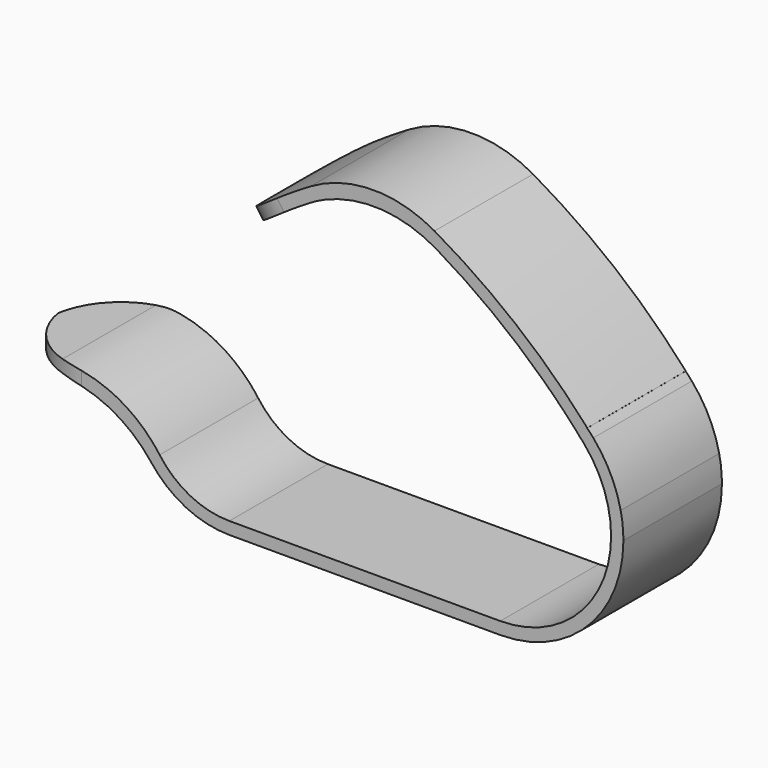
from build123d import *

# Parameters (mm, degrees)
F1_DEPTH    = 5
F2_R        = 5
F3_R        = 5
F4_R        = 5
F5_R        = 5
F6_R        = 2.49999
F7_T1_DEPTH = 15.5


# Not quite as in the source:
# - a fillet or chamfer that OpenCascade refuses, or shapes differently, is made with other operations: its cross-section is extruded or revolved along the edge and cut away or added
# - a fillet or chamfer is up to 0.001 mm smaller than in the source, because OpenCascade refuses the exact size
# - ends of sketch curves that miss each other by under 0.0002 mm in the source are joined


with BuildPart() as f1:
    # F0 (on Front) → F1 (new body)
    with BuildSketch(Plane.XZ):
        with BuildLine():
            ThreePointArc((8.5340575526, 1.5524331459), (5.288604189, 4.5896124098), (1.5539747452, 7))
            Line((1.5539747452, 7), (0.4354276506, 7))
            ThreePointArc((0.4354276506, 7), (3.7532215697, 5.0934578086), (6.7313555625, 2.6906724375))
            ThreePointArc((6.7313555625, 2.6906724375), (7.6907583635, 2.2142400773), (8.526661649, 1.544383954))
            Line((8.526661649, 1.544383954), (8.5340575526, 1.5524331459))
        make_face()
        with BuildLine():
            Line((0.4354276506, 7), (1.5539747452, 7))
            ThreePointArc((1.5539747452, 7), (0.9960319704, 7.2841112302), (0.4311083103, 7.5540752821))
            ThreePointArc((0.4311083103, 7.5540752821), (0.1227273169, 7.4207378189), (-0.1837962437, 7.2831841097))
            ThreePointArc((-0.1837962437, 7.2831841097), (0.1268056153, 7.1437566434), (0.4354276506, 7))
        make_face()
        with BuildLine():
            ThreePointArc((-0.1837962437, 7.2831841097), (0.1227273169, 7.4207378189), (0.4311083103, 7.5540752821))
            ThreePointArc((0.4311083103, 7.5540752821), (0.1226739578, 7.6941799666), (-0.1876416897, 7.830066947))
            ThreePointArc((-0.1876416897, 7.830066947), (-0.4960575858, 7.6899267332), (-0.8025462438, 7.5456202987))
            ThreePointArc((-0.8025462438, 7.5456202987), (-0.4922657174, 7.4165371782), (-0.1837962437, 7.2831841097))
        make_face()
        with BuildLine():
            ThreePointArc((9.8891323912, -0.952916211), (9.474622014, 0.231088934), (8.7784454506, 1.2746526497))
            ThreePointArc((8.7784454506, 1.2746526497), (8.6550425686, 1.4118417052), (8.526661649, 1.544383954))
            Line((8.526661649, 1.544383954), (8.1941180403, 1.1824664061))
            ThreePointArc((8.1941180403, 1.1824664061), (8.2977627182, 1.0651806637), (8.4006513445, 0.9472311186))
            ThreePointArc((8.4006513445, 0.9472311186), (9.1684512833, 0.0156127298), (9.8891323912, -0.952916211))
        make_face()
        with BuildLine():
            ThreePointArc((-5.7758389138, 3.7449434933), (-3.3782514437, 5.5249211523), (-0.7819293264, 7))
            Line((-0.7819293264, 7), (-1.874342087, 7))
            ThreePointArc((-1.874342087, 7), (-4.0392081747, 5.6857592036), (-6.0600011216, 4.1592370405))
            Line((-6.0600011216, 4.1592370405), (-5.7758389138, 3.7449434933))
        make_face()
        with BuildLine():
            Line((-1.874342087, 7), (-0.7819293264, 7))
            ThreePointArc((-0.7819293264, 7), (-0.4838189836, 7.143611709), (-0.1837962437, 7.2831841097))
            ThreePointArc((-0.1837962437, 7.2831841097), (-0.4922657174, 7.4165371782), (-0.8025462438, 7.5456202987))
            ThreePointArc((-0.8025462438, 7.5456202987), (-1.341725683, 7.2792562383), (-1.874342087, 7))
        make_face()
        with BuildLine():
            ThreePointArc((8.526661649, 1.544383954), (7.6907583635, 2.2142400773), (6.7313555625, 2.6906724375))
            ThreePointArc((6.7313555625, 2.6906724375), (7.4790116412, 1.9523538866), (8.1941180403, 1.1824664061))
            Line((8.1941180403, 1.1824664061), (8.526661649, 1.544383954))
        make_face()
        with BuildLine():
            ThreePointArc((5, -7), (8.5355339059, -5.5355339059), (10, -2))
            ThreePointArc((10, -2), (9.9722058463, -1.4735315565), (9.8891323912, -0.952916211))
            ThreePointArc((9.8891323912, -0.952916211), (9.1684512833, 0.0156127298), (8.4006513445, 0.9472311186))
            ThreePointArc((8.4006513445, 0.9472311186), (9.2162011355, -0.4272164851), (9.5, -2))
            ThreePointArc((9.5, -2), (8.1819805153, -5.1819805153), (5, -6.5))
            Line((5, -6.5), (5, -7))
        make_face()
        with BuildLine():
            Line((4.8047364689, -6.5), (2.8205505282, -6.5))
            ThreePointArc((2.8205505282, -6.5), (3.7870014268, -6.8506323775), (4.8047364689, -6.9961857605))
            Line((4.8047364689, -6.9961857605), (4.8047364689, -6.5))
        make_face()
        with BuildLine():
            ThreePointArc((4.8047364689, -6.9961857605), (3.7870014268, -6.8506323775), (2.8205505282, -6.5))
            Line((2.8205505282, -6.5), (-4.0635083269, -6.5))
            ThreePointArc((-4.0635083269, -6.5), (-5, -6.8729833462), (-6, -7))
            Line((-6, -7), (4.8047364689, -7))
            Line((4.8047364689, -7), (4.8047364689, -6.9961857605))
        make_face()
        with BuildLine():
            ThreePointArc((8.4006513445, 0.9472311186), (8.2977627182, 1.0651806637), (8.1941180403, 1.1824664061))
            Line((8.1941180403, 1.1824664061), (8.1880677147, 1.1758816487))
            ThreePointArc((8.1880677147, 1.1758816487), (8.2963182158, 1.0633782366), (8.4006513445, 0.9472311186))
        make_face()
        with BuildLine():
            ThreePointArc((4.8047364689, -6.9961857605), (4.9023496096, -6.9990463492), (5, -7))
            Line((5, -7), (5, -6.5))
            Line((5, -6.5), (4.8047364689, -6.5))
            Line((4.8047364689, -6.5), (4.8047364689, -6.9961857605))
        make_face()
        with BuildLine():
            ThreePointArc((-6, -7), (-5, -6.8729833462), (-4.0635083269, -6.5))
            Line((-4.0635083269, -6.5), (-6, -6.5))
            Line((-6, -6.5), (-6, -7))
        make_face()
        with BuildLine():
            Line((-12.1979728804, -3.5), (-11.6333076528, -3.5))
            ThreePointArc((-11.6333076528, -3.5), (-11.4981121732, -3.2492054316), (-11.3600093633, -3))
            Line((-11.3600093633, -3), (-11.9317121995, -3))
            ThreePointArc((-11.9317121995, -3), (-12.0662587747, -3.2492458247), (-12.1979728804, -3.5))
        make_face()
        with BuildLine():
            ThreePointArc((-11.3600093633, -3), (-11.4981121732, -3.2492054316), (-11.6333076528, -3.5))
            Line((-11.6333076528, -3.5), (-10, -3.5))
            Line((-10, -3.5), (-10, -3))
            Line((-10, -3), (-11.3600093633, -3))
        make_face()
        with BuildLine():
            ThreePointArc((-9.9686269666, -3.5), (-9.9921490369, -3.2504916502), (-10, -3))
            Line((-10, -3), (-10, -3.5))
            Line((-10, -3.5), (-9.9686269666, -3.5))
        make_face()
        with BuildLine():
            Line((-9.5, -3), (-10, -3))
            ThreePointArc((-10, -3), (-9.9921490369, -3.2504916502), (-9.9686269666, -3.5))
            Line((-9.9686269666, -3.5), (-9.4641016151, -3.5))
            ThreePointArc((-9.4641016151, -3.5), (-9.491013868, -3.2506435188), (-9.5, -3))
        make_face()
        with BuildLine():
            ThreePointArc((-9.9686269666, -3.5), (-8.6457513111, -6), (-6, -7))
            Line((-6, -7), (-6, -6.5))
            ThreePointArc((-6, -6.5), (-8.2912878475, -5.6457513111), (-9.4641016151, -3.5))
            Line((-9.4641016151, -3.5), (-9.9686269666, -3.5))
        make_face()
        with BuildLine():
            Line((-15, -3.5), (-12.1979728804, -3.5))
            ThreePointArc((-12.1979728804, -3.5), (-12.0662587747, -3.2492458247), (-11.9317121995, -3))
            Line((-11.9317121995, -3), (-15, -3))
            Line((-15, -3), (-15, -3.5))
        make_face()
    extrude(amount=F1_DEPTH)

    # F2
    f2_edges = [f1.edges().sort_by_distance(p)[0] for p in [
        (-9.968627, -2.5, -3.5),
    ]]
    fillet(f2_edges, radius=F2_R)

    # F3
    f3_edges = [f1.edges().sort_by_distance(p)[0] for p in [
        (-9.5, -2.5, -3),
    ]]
    fillet(f3_edges, radius=F3_R)

    # F4
    f4_edges = [f1.edges().sort_by_distance(p)[0] for p in [
        (-0.183796, -2.5, 7.283184),
    ]]
    fillet(f4_edges, radius=F4_R)

    # F5
    f5_edges = [f1.edges().sort_by_distance(p)[0] for p in [
        (-0.187642, -2.5, 7.830067),
    ]]
    fillet(f5_edges, radius=F5_R)

    # F6 (radius 2.5 in the source; OpenCascade refuses exactly that, so slightly less here)
    f6_edges = [f1.edges().sort_by_distance(p)[0] for p in [
        (-5.91792, -5, 3.95209),
        (-5.91792, 0, 3.95209),
    ]]
    fillet(f6_edges, radius=F6_R)

    # F7: fillet of radius 3 on 2 edges, made by hand

    # F7_s2 → F7_t1 (cut)
    with BuildSketch(Plane.XY.offset(-11)):
        with BuildLine():
            ThreePointArc((-15, -2), (-14.1213203436, -4.1213203436), (-12, -5))
            Line((-12, -5), (-15, -5))
            Line((-15, -5), (-15, -2))
        make_face()
        with BuildLine():
            ThreePointArc((-12, 0), (-14.1213203436, -0.8786796564), (-15, -3))
            Line((-15, -3), (-15, 0))
            Line((-15, 0), (-12, 0))
        make_face()
    extrude(amount=F7_T1_DEPTH, mode=Mode.SUBTRACT)


solid = f1.part
